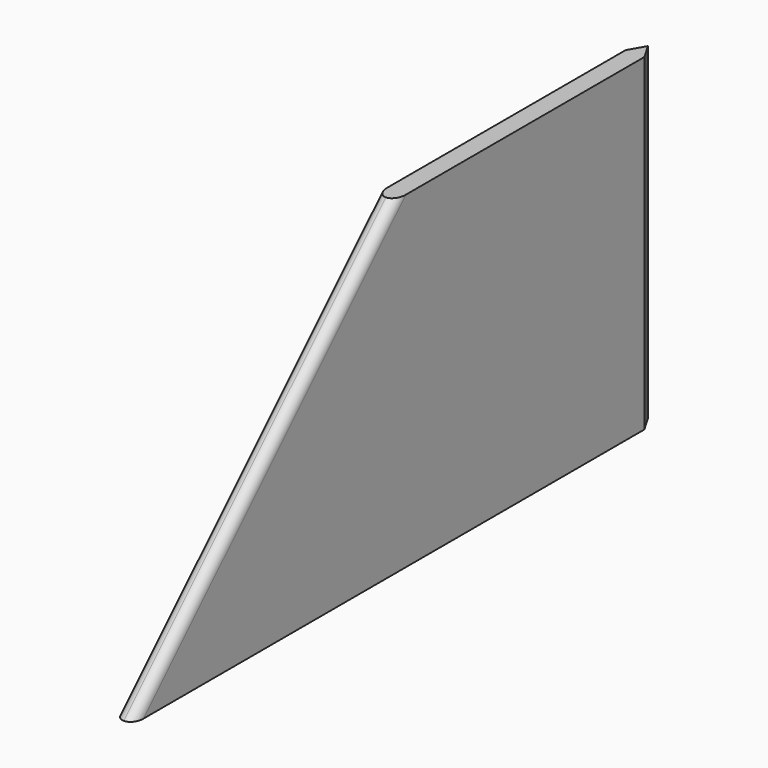
from build123d import *

# Parameters (mm, degrees)
F0_W     = 70
F0_H     = 5
F1_DEPTH = 1
F2_R     = 1
F3_R     = 0.99999
F5_DEPTH = 75
F6_SIZE2 = 1.7320508076
F6_SIZE  = 1
F7_SIZE2 = 1.732041
F7_SIZE  = 0.99999


# Not quite as in the source:
# - a fillet or chamfer is up to 0.001 mm smaller than in the source, because OpenCascade refuses the exact size


with BuildPart() as f1:
    # F0 (on Right) → F1 (new body, symmetric)
    with BuildSketch(Plane.YZ):
        Polygon((-70, 0), (0, 0), (0, 35), (-35, 35), align=None)
        with Locations((-35, -2.5)):
            Rectangle(F0_W, F0_H)
    extrude(amount=F1_DEPTH, both=True)

    # F2
    f2_edges = [f1.edges().sort_by_distance(p)[0] for p in [
        (1, -52.5, 17.5),
    ]]
    fillet(f2_edges, radius=F2_R)

    # F3 (radius 1 in the source; OpenCascade refuses exactly that, so slightly less here)
    f3_edges = [f1.edges().sort_by_distance(p)[0] for p in [
        (-1, -52.5, 17.5),
    ]]
    fillet(f3_edges, radius=F3_R)

    # F4 (on Front) → F5 (cut, symmetric)
    with BuildSketch(Plane.XZ):
        with BuildLine():
            ThreePointArc((0, 0), (-11.6672618896, -28.1672618896), (16.5, -16.5))
            ThreePointArc((16.5, -16.5), (11.6672618896, -4.8327381104), (0, 0))
        make_face()
    extrude(amount=F5_DEPTH, both=True, mode=Mode.SUBTRACT)

    # F6
    f6_edges = [f1.edges().sort_by_distance(p)[0] for p in [
        (1, 0, 17.484835),
    ]]
    f6_side = f1.faces().sort_by_distance((0, 0, 17.494946))[0]
    chamfer(f6_edges, length=F6_SIZE, length2=F6_SIZE2, reference=f6_side)

    # F7 (size 1 and 1.7320508076 in the source; OpenCascade refuses exactly that, so slightly less here)
    f7_edges = [f1.edges().sort_by_distance(p)[0] for p in [
        (-1, 0, 17.484835),
    ]]
    f7_side = f1.faces().sort_by_distance((-0.500072, 0, 17.494946))[0]
    chamfer(f7_edges, length=F7_SIZE, length2=F7_SIZE2, reference=f7_side)


solid = f1.part
